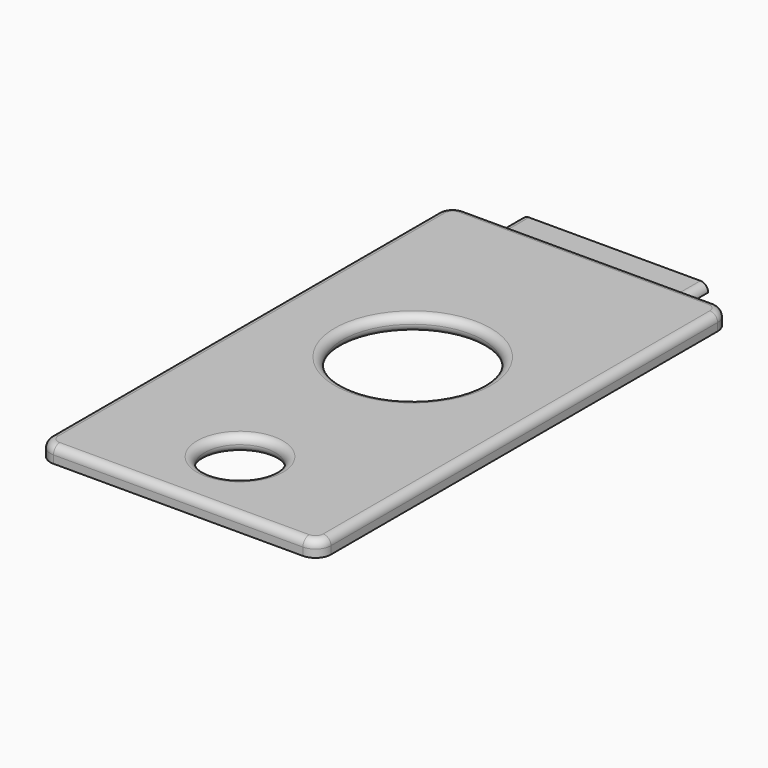
from build123d import *

# Parameters (mm, degrees)
F0_R     = 2.25
F0_R_2   = 4.5
F1_DEPTH = 1
F2_R     = 0.5
F0_W     = 12
F0_H     = 2
F3_DEPTH = 0.5
F4_R     = 0.49999
F5_R     = 0.49999


# Not quite as in the source:
# - a fillet or chamfer is up to 0.001 mm smaller than in the source, because OpenCascade refuses the exact size


with BuildPart() as f1:
    # F0 (on Top) → F1 (new body)
    with BuildSketch(Plane.XY):
        with BuildLine():
            ThreePointArc((-2, -1), (-1.7071067812, -1.7071067812), (-1, -2))
            Line((-1, -2), (15, -2))
            ThreePointArc((15, -2), (15.7071067812, -1.7071067812), (16, -1))
            Line((16, -1), (16, 30))
            ThreePointArc((16, 30), (15.7071067812, 30.7071067812), (15, 31))
            Line((15, 31), (13, 31))
            Line((13, 31), (1, 31))
            Line((1, 31), (-1, 31))
            ThreePointArc((-1, 31), (-1.7071067812, 30.7071067812), (-2, 30))
            Line((-2, 30), (-2, -1))
        make_face()
        with Locations((7, 2.95)):
            Circle(F0_R, mode=Mode.SUBTRACT)
        with Locations((7, 16.8)):
            Circle(F0_R_2, mode=Mode.SUBTRACT)
    extrude(amount=F1_DEPTH)

    # F2
    f2_edges = [f1.edges().sort_by_distance(p)[0] for p in [
        (2.5, 16.8, 0),
        (4.75, 2.95, 0),
    ]]
    fillet(f2_edges, radius=F2_R)

    # F0 (on Top) → F3 (join)
    with BuildSketch(Plane.XY):
        with Locations((7, 32)):
            Rectangle(F0_W, F0_H)
    extrude(amount=F3_DEPTH)

    # F4 (radius 0.5 in the source; OpenCascade refuses exactly that, so slightly less here)
    f4_edges = [f1.edges().sort_by_distance(p)[0] for p in [
        (-2, 14.5, 1),
        (-1.707107, -1.707107, 1),
        (7, -2, 1),
        (15.707107, -1.707107, 1),
        (16, 14.5, 1),
        (15.707107, 30.707107, 1),
        (7, 31, 1),
        (-1.707107, 30.707107, 1),
        (4.75, 2.95, 1),
        (2.5, 16.8, 1),
    ]]
    fillet(f4_edges, radius=F4_R)

    # F5 (radius 0.5 in the source; OpenCascade refuses exactly that, so slightly less here)
    f5_edges = [f1.edges().sort_by_distance(p)[0] for p in [
        (1, 32, 0.5),
        (13, 32, 0.5),
    ]]
    fillet(f5_edges, radius=F5_R)


solid = f1.part
